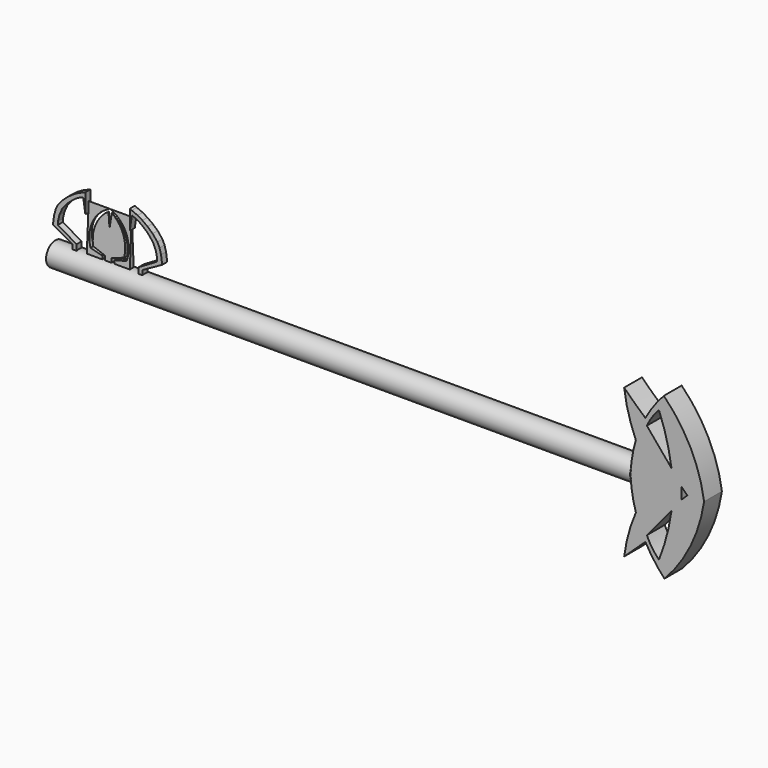
from build123d import *

# Parameters (mm, degrees)
F0_R        = 5.5929426232
F1_DEPTH    = 279.4
F5_DEPTH    = 1.4986
F6_DEPTH    = 5.334
F7_DEPTH    = 1.778
F8_T1_DEPTH = 192.2731836011
F10_DEPTH   = 12.7


# Not quite as in the source:
# - a fillet or chamfer that OpenCascade refuses, or shapes differently, is made with other operations: its cross-section is extruded or revolved along the edge and cut away or added


with BuildPart() as f1:
    # F0 (on Right) → F1 (new body)
    with BuildSketch(Plane.YZ):
        Circle(F0_R)
    extrude(amount=-F1_DEPTH)

    # F2 (on Front) → F5 (join, symmetric)
    with BuildSketch(Plane.XZ):
        Polygon((-278.8294255733, 16.9219542295), (-279.4027328491, 12.8565793857), (-270.0211107731, 7.6445620507), (-270.0211107731, 5.6118746288), (-270.0211107731, 0), (-236.3921552896, 0), (-236.4905774593, 5.6118746288), (-236.4905774593, 7.6445620507), (-227.1089553833, 12.8565793857), (-227.6822626591, 16.9219542295), (-228.4119427204, 19.5800829679), (-229.402244091, 21.7170100659), (-231.692014207, 24.531500414), (-234.1451644897, 26.7205480486), (-236.594825983, 28.4926332533), (-238.8881146908, 29.8477597535), (-241.6504919529, 31.0465227813), (-242.6407635212, 31.4634852111), (-242.6407635212, 22.1339724958), (-241.6009604931, 28.9600603282), (-238.8881146908, 27.8671924025), (-236.2821102142, 25.9387455881), (-234.0409457684, 24.0102987736), (-231.5391600132, 20.9352076054), (-230.1840484142, 17.7558772266), (-229.5064926147, 14.8371467367), (-229.5064926147, 13.4299015626), (-238.4190261364, 8.1657636911), (-238.4190261364, 5.6639946997), (-238.4190261364, 1.6877186717), (-268.2300508022, 1.6877186717), (-268.092662096, 5.6639946997), (-268.092662096, 8.1657636911), (-277.0051956177, 13.4299015626), (-277.0051956177, 14.8371467367), (-276.3276398182, 17.7558772266), (-274.9725282192, 20.9352076054), (-272.4707424641, 24.0102987736), (-270.2295780182, 25.9387455881), (-267.6235735416, 27.8671924025), (-264.9107277393, 28.9600603282), (-263.8709247112, 22.1339724958), (-263.8709247112, 31.4634852111), (-264.8611962795, 31.0465227813), (-267.6235735416, 29.8477597535), (-269.9168622494, 28.4926332533), (-272.3665237427, 26.7205480486), (-274.8196740255, 24.531500414), (-277.1094441414, 21.7170100659), (-278.099745512, 19.5800829679), align=None)
    extrude(amount=F5_DEPTH, both=True)

    # F3 (on Front) → F6 (join, symmetric)
    with BuildSketch(Plane.XZ):
        with BuildLine():
            ThreePointArc((0.0101553228, 0.2840123077), (-0.0967004528, 0.1418930692), (-0.2038563749, 0))
            Line((-0.2038563749, 0), (0, 0))
            ThreePointArc((0, 0), (0.0049059903, 0.1420122922), (0.0101553228, 0.2840123077))
        make_face()
        with BuildLine():
            Line((0, 0), (-0.2038563749, 0))
            ThreePointArc((-0.2038563749, 0), (-0.0966486695, -0.1433570013), (0.0102668641, -0.2869320359))
            ThreePointArc((0.0102668641, -0.2869320359), (0.004958213, -0.1434722876), (0, 0))
        make_face()
        with BuildLine():
            ThreePointArc((0.0101553228, 0.2840123077), (0.0049059903, 0.1420122922), (0, 0))
            ThreePointArc((0, 0), (0.004958213, -0.1434722876), (0.0102668641, -0.2869320359))
            ThreePointArc((0.0102668641, -0.2869320359), (0.7907915752, -7.8454061019), (2.54, -15.24))
            Line((2.54, -15.24), (2.54, 15.24))
            ThreePointArc((2.54, 15.24), (0.7905478985, 7.8439656383), (0.0101553228, 0.2840123077))
        make_face()
        with BuildLine():
            Line((2.54, 15.24), (2.54, -15.24))
            ThreePointArc((2.54, -15.24), (4.5439363149, -20.7794421559), (7.0923387837, -26.0904519478))
            ThreePointArc((7.0923387837, -26.0904519478), (11.2408564011, -32.6543576843), (16.2185082823, -38.6140589091))
            Line((16.2185082823, -38.6140589091), (23.6472193128, -6.1149669525))
            Line((23.6472193128, -6.1149669525), (19.8538427248, 0))
            Line((19.8538427248, 0), (23.928701104, 5.9311091676))
            Line((23.928701104, 5.9311091676), (15.9117437896, 38.290112876))
            ThreePointArc((15.9117437896, 38.290112876), (11.1082726784, 32.4716804641), (7.0898126318, 26.0858))
            ThreePointArc((7.0898126318, 26.0858), (4.5429123731, 20.7770014472), (2.54, 15.24))
        make_face()
        with BuildLine():
            ThreePointArc((19.5732042193, -8.9976880699), (17.2672693148, -20.4441869398), (13.5875111446, -31.5256603062))
            ThreePointArc((13.5875111446, -31.5256603062), (10.3065645811, -27.5541885084), (7.7893436652, -23.0596587829))
            Line((7.7893436652, -23.0596587829), (19.5732042193, -8.9976880699))
        make_face(mode=Mode.SUBTRACT)
        with BuildLine():
            Line((19.5732042193, 8.9976880699), (7.7893436652, 23.0596587829))
            ThreePointArc((7.7893436652, 23.0596587829), (10.3065645811, 27.5541885084), (13.5875111446, 31.5256603062))
            ThreePointArc((13.5875111446, 31.5256603062), (17.2672693148, 20.4441869398), (19.5732042193, 8.9976880699))
        make_face(mode=Mode.SUBTRACT)
        with BuildLine():
            ThreePointArc((7.0923387837, -26.0904519478), (4.5439363149, -20.7794421559), (2.54, -15.24))
            ThreePointArc((2.54, -15.24), (-0.9901478251, -25.1995599957), (-3.0676612163, -35.56))
            Line((-3.0676612163, -35.56), (7.0923387837, -26.0904519478))
        make_face()
        with BuildLine():
            ThreePointArc((-3.0701873682, 35.56), (-0.9914342988, 25.1994632411), (2.54, 15.24))
            ThreePointArc((2.54, 15.24), (4.5429123731, 20.7770014472), (7.0898126318, 26.0858))
            ThreePointArc((7.0898126318, 26.0858), (1.9231383714, 30.7299517315), (-3.0701873682, 35.56))
        make_face()
        with BuildLine():
            Line((23.6472193128, -6.1149669525), (16.2185082823, -38.6140589091))
            ThreePointArc((16.2185082823, -38.6140589091), (28.6827408005, -20.7741612342), (35.1675897837, 0))
            ThreePointArc((35.1675897837, 0), (28.6506436465, 20.709546245), (15.9117437896, 38.290112876))
            Line((15.9117437896, 38.290112876), (23.928701104, 5.9311091676))
            Line((23.928701104, 5.9311091676), (19.8538427248, 0))
            Line((19.8538427248, 0), (23.6472193128, -6.1149669525))
        make_face()
        Polygon((24.3763010949, 2.7386606671), (27.1741487086, 0), (24.3763010949, -2.7386606671), align=None, mode=Mode.SUBTRACT)
    extrude(amount=F6_DEPTH, both=True)


with BuildPart() as f7:
    # F4 (on Front) → F7 (new body, symmetric)
    with BuildSketch(Plane.XZ):
        Polygon((-263.461381197, 22.2413148731), (-263.461381197, 5.6046764366), (-243.5538172722, 5.6046764366), (-242.8830116987, 5.6046764366), (-242.8830116987, 27.2857323289), (-263.461381197, 27.2857323289), align=None)
    extrude(amount=F7_DEPTH, both=True)

    # F8: chamfer of 1.778 x 33.02 on 2 edges, made by hand

    # F8_s2 → F8_t1 (cut)
    with BuildSketch(Plane.YZ.offset(-349.3087882484)):
        Polygon((0, 27.2857323289), (-1.778, -5.7342676711), (-1.778, 27.2857323289), align=None)
        Polygon((1.778, -5.7342676711), (0, 27.2857323289), (1.778, 27.2857323289), align=None)
    extrude(amount=F8_T1_DEPTH, mode=Mode.SUBTRACT)

    # F9 (on face) → F10 (cut, symmetric)
    with BuildSketch(Plane(origin=(0, -1.4649841536, 0.0788837621), x_dir=(1, 0, 0), z_dir=(0, -0.9985534407, 0.0537682622))):
        with BuildLine():
            Line((-253.9569606738, 25.8916511639), (-253.1721964478, 19.1923287956))
            Line((-253.1721964478, 19.1923287956), (-253.1721964478, 27.2462618997))
            ThreePointArc((-253.1721964478, 27.2462618997), (-261.2199041562, 19.5756184054), (-261.8029889563, 8.4731689868))
            Line((-261.8029889563, 8.4731689868), (-256.0348063707, 7.0519491145))
            Line((-256.0348063707, 7.0519491145), (-256.0348063707, 5.5337976408))
            Line((-256.0348063707, 5.5337976408), (-254.723623395, 5.5337976408))
            Line((-254.723623395, 5.5337976408), (-254.723623395, 7.4541432704))
            Line((-254.723623395, 7.4541432704), (-260.5685285915, 9.5231209762))
            ThreePointArc((-260.5685285915, 9.5231209762), (-259.7972246978, 18.731111896), (-253.9569606738, 25.8916511639))
        make_face()
        with BuildLine():
            Line((-251.6207695007, 7.4541432704), (-251.6207695007, 5.5337976408))
            Line((-251.6207695007, 5.5337976408), (-250.309586525, 5.5337976408))
            Line((-250.309586525, 5.5337976408), (-250.309586525, 7.0519491145))
            Line((-250.309586525, 7.0519491145), (-244.5414039394, 8.4731689868))
            ThreePointArc((-244.5414039394, 8.4731689868), (-245.1244887395, 19.5756184054), (-253.1721964478, 27.2462618997))
            Line((-253.1721964478, 27.2462618997), (-253.1721964478, 19.1923287956))
            Line((-253.1721964478, 19.1923287956), (-252.3874322219, 25.8916511639))
            ThreePointArc((-252.3874322219, 25.8916511639), (-246.5471681979, 18.731111896), (-245.7758643042, 9.5231209762))
            Line((-245.7758643042, 9.5231209762), (-251.6207695007, 7.4541432704))
        make_face()
    extrude(amount=F10_DEPTH, both=True, mode=Mode.SUBTRACT)


solid = Compound([f1.part, f7.part])
